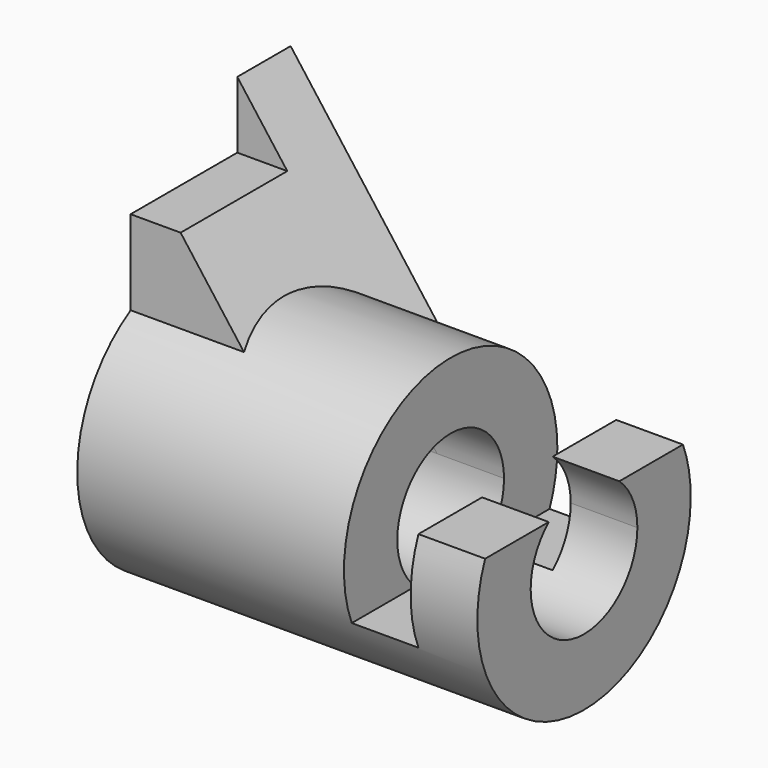
from build123d import *
from build123d import SkipClean  # not in build123d's __all__

# Parameters (mm, degrees)
F0_R          = 25.4
F0_R_2        = 12.7
F1_DEPTH      = 76.2
F3_DEPTH      = 26.67
F5_DEPTH      = 12.7
F5_DEPTH_BACK = 25.4
F6_W          = 25.4
F6_H          = 12.7
F7_DEPTH      = 76.201
F8_R          = 12.7
F9_DEPTH      = 76.201


with BuildPart() as f1:
    # F0 (on Right) → F1 (new body)
    with BuildSketch(Plane.YZ):
        Circle(F0_R)
        Circle(F0_R_2, mode=Mode.SUBTRACT)
    extrude(amount=F1_DEPTH)

    # F2 (on Front) → F3 (cut, symmetric)
    with BuildSketch(Plane.XZ):
        Polygon((76.2, 25.4), (50.8, 25.4), (50.8, -9.525), (63.5, -9.525), (63.5, 9.525), (76.2, 9.525), align=None)
    extrude(amount=F3_DEPTH, both=True, mode=Mode.SUBTRACT)

    # F4 (on Front) → F5 (join, two sides)
    with BuildSketch(Plane.XZ) as f5_sk:
        Polygon((0, 50.8), (0, 0), (38.1, 0), align=None)
    extrude(amount=F5_DEPTH)
    extrude(f5_sk.sketch, amount=-F5_DEPTH_BACK)

    # F6 (on face) → F7 (cut, through all)
    with BuildSketch(Plane(origin=(0, 0, 0), x_dir=(0, -1, 0), z_dir=(-1, 0, 0))):
        with Locations((0, 44.45)):
            Rectangle(F6_W, F6_H)
    extrude(amount=-F7_DEPTH, mode=Mode.SUBTRACT)

    # F8 (on face) → F9 (cut, through all)
    with BuildSketch(Plane(origin=(0, 0, 0), x_dir=(0, -1, 0), z_dir=(-1, 0, 0))):
        Circle(F8_R)
    with SkipClean():  # cleaning this boolean's faces spoils the solid; the shape is the same uncleaned
        extrude(amount=-F9_DEPTH, mode=Mode.SUBTRACT)


solid = f1.part
